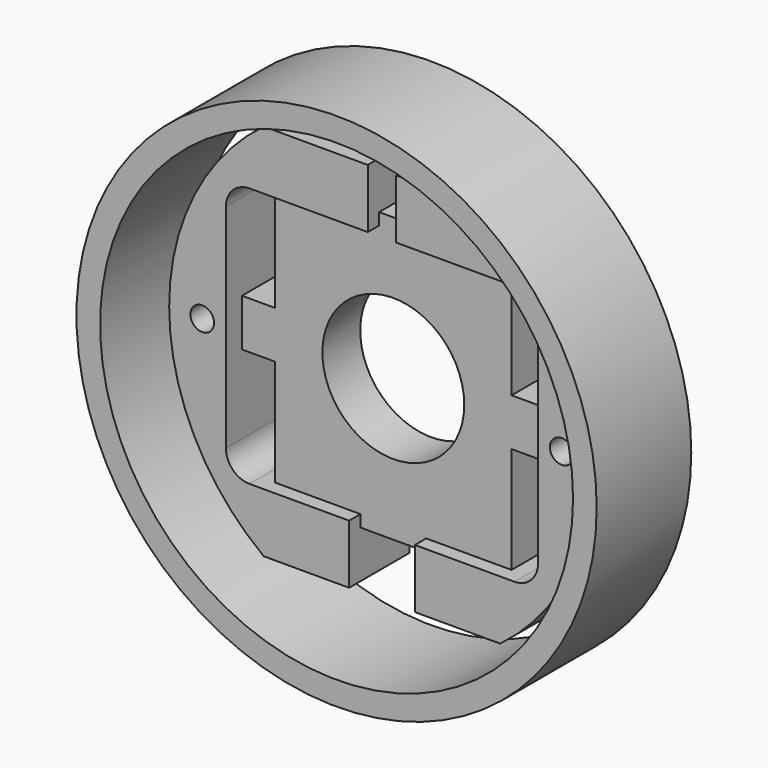
from build123d import *

# Parameters (mm, degrees)
F0_W          = 50
F0_H          = 60
F0_R          = 15
F1_DEPTH      = 10
F2_R          = 2.5
F3_DEPTH      = 13
F3_DEPTH_BACK = 3
F4_W          = 10
F4_H          = 10
F5_DEPTH      = 7
F7_R          = 55
F7_R_2        = 50
F8_DEPTH      = 25


# Not quite as in the source:
# - a feature names something its author has since deleted; it is built from what else it names


with BuildPart() as f1:
    # F0 (on Front) → F1 (new body)
    with BuildSketch(Plane.XZ):
        Rectangle(F0_W, F0_H)
        Circle(F0_R, mode=Mode.SUBTRACT)
    extrude(amount=F1_DEPTH)

    # F2 (on Front) → F3 (join, two sides)
    with BuildSketch(Plane.XZ) as f3_sk:
        with BuildLine():
            Line((-3, 40), (-25, 40))
            ThreePointArc((-25, 40), (-45, 0), (-25, -40))
            Line((-25, -40), (-6.9549679495, -40))
            Line((-6.9549679495, -40), (-6.9549679495, -27.5))
            Line((-6.9549679495, -27.5), (-28, -27.5))
            ThreePointArc((-28, -27.5), (-31.5355339059, -26.0355339059), (-33, -22.5))
            Line((-33, -22.5), (-33, 22.5))
            ThreePointArc((-33, 22.5), (-31.5355339059, 26.0355339059), (-28, 27.5))
            Line((-28, 27.5), (-3, 27.5))
            Line((-3, 27.5), (-3, 40))
        make_face()
        with Locations((-38, 0)):
            Circle(F2_R, mode=Mode.SUBTRACT)
    extrude(amount=F3_DEPTH)
    extrude(f3_sk.sketch, amount=-F3_DEPTH_BACK)

    # F4 (on face) → F5 (join)
    with BuildSketch(Plane(origin=(-25, 0, 0), x_dir=(0, -1, 0), z_dir=(-1, 0, 0))):
        with Locations((5, 0)):
            Rectangle(F4_W, F4_H)
    extrude(amount=F5_DEPTH)

    # F6: F1 across plane


with BuildPart() as f1_1:
    add(f1.part)
    add(f1.part.mirror(Plane.YZ))


with BuildPart() as f8:
    # F7 (on Front) → F8 (new body)
    with BuildSketch(Plane.XZ):
        Circle(F7_R)
        Circle(F7_R_2, mode=Mode.SUBTRACT)
    extrude(amount=F8_DEPTH)


solid = Compound([f1_1.part, f8.part])
